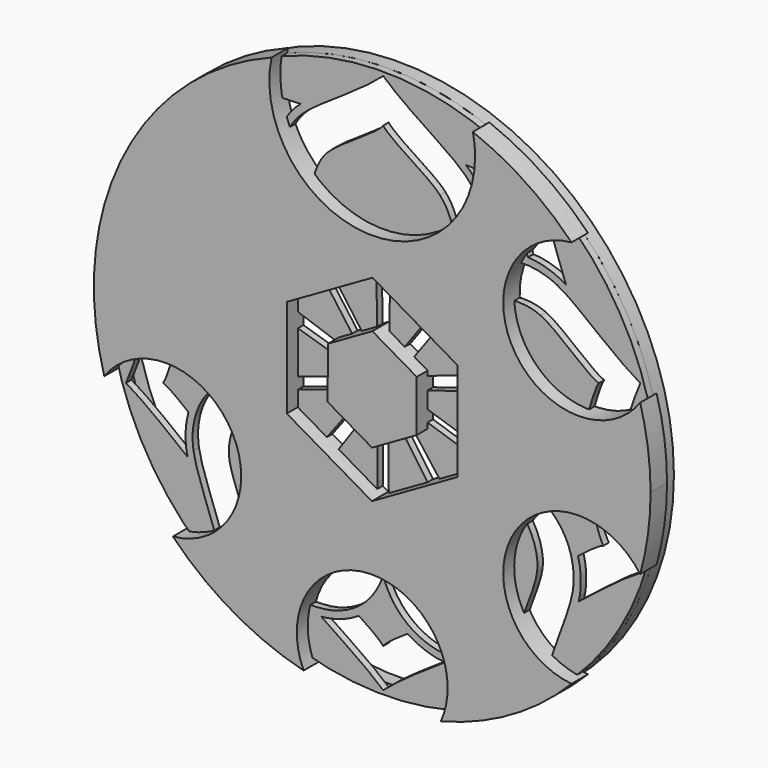
from build123d import *

# Parameters (mm, degrees)
F0_R     = 40
F1_DEPTH = 1
F2_R     = 40
F3_DEPTH = 2
F4_T     = -1
F6_DEPTH = 3


with BuildPart() as f1:
    # F0 (on Front) → F1 (new body)
    with BuildSketch(Plane.XZ):
        Circle(F0_R)
        with BuildLine():
            add(Edge.make_bspline(
                [(3.5534648058, -31.0212486438), (5.4467639917, -32.2635820829), (7.3085112664, -32.6879645142), (8.144360142, -32.8156482718)],
                knots=[0, 0, 0, 0, 1, 1, 1, 1], degree=3))
            add(Edge.make_bspline(
                [(8.144360142, -32.8156482718), (8.4174410108, -32.8579020009), (8.7100803743, -32.889269398), (9.012129957, -32.9147323438)],
                knots=[0, 0, 0, 0, 1, 1, 1, 1], degree=3))
            add(Edge.make_bspline(
                [(9.012129957, -32.9147323438), (6.2822438391, -34.821316545), (2.7349602557, -36.9727509576), (-0.0059967083, -39.430109749)],
                knots=[0, 0, 0, 0, 1, 1, 1, 1], degree=3))
            add(Edge.make_bspline(
                [(-0.0059967083, -39.430109749), (-2.7493523555, -36.969798732), (-6.3001417068, -34.8165191784), (-9.0315039375, -32.9086433785)],
                knots=[0, 0, 0, 0, 1, 1, 1, 1], degree=3))
            add(Edge.make_bspline(
                [(-9.0315039375, -32.9086433785), (-8.7255795588, -32.8831804326), (-8.4292499133, -32.8518130356), (-8.153585847, -32.8099283347)],
                knots=[0, 0, 0, 0, 1, 1, 1, 1], degree=3))
            Line((-8.153585847, -32.8099283347), (-8.1548774457, -32.8093747924))
            add(Edge.make_bspline(
                [(-8.1548774457, -32.8093747924), (-7.3169989151, -32.6818755489), (-5.4502697596, -32.2654272239), (-3.5521732071, -31.0286292078)],
                knots=[0, 0, 0, 0, 1, 1, 1, 1], degree=3))
            add(Edge.make_bspline(
                [(-3.5521732071, -31.0286292078), (-2.0007786495, -32.048992184), (-0.5704253419, -33.0138164159), (-0.0059967083, -33.7646042911)],
                knots=[0, 0, 0, 0, 1, 1, 1, 1], degree=3))
            add(Edge.make_bspline(
                [(-0.0059967083, -33.7646042911), (0.5611996369, -33.0114177325), (1.996165797, -32.0441948174), (3.5534648058, -31.0212486438)],
                knots=[0, 0, 0, 0, 1, 1, 1, 1], degree=3))
        make_face(mode=Mode.SUBTRACT)
        with BuildLine():
            add(Edge.make_bspline(
                [(-28.4049309548, -12.9656213328), (-29.0009114997, -15.1502682835), (-28.8293133861, -17.0520551181), (-28.6925884376, -17.8864278808)],
                knots=[0, 0, 0, 0, 1, 1, 1, 1], degree=3))
            add(Edge.make_bspline(
                [(-28.6925884376, -17.8864278808), (-28.649227624, -18.1589552074), (-28.5875999144, -18.4467972042), (-28.5185916408, -18.7416507369)],
                knots=[0, 0, 0, 0, 1, 1, 1, 1], degree=3))
            add(Edge.make_bspline(
                [(-28.5185916408, -18.7416507369), (-31.1759637171, -16.7352444074), (-34.3184233639, -14.026577411), (-37.501845141, -12.1792222362)],
                knots=[0, 0, 0, 0, 1, 1, 1, 1], degree=3))
            add(Edge.make_bspline(
                [(-37.501845141, -12.1792222362), (-36.0098641238, -8.8094412175), (-35.0594319918, -4.76655276), (-34.0887033087, -1.5801787573)],
                knots=[0, 0, 0, 0, 1, 1, 1, 1], degree=3))
            add(Edge.make_bspline(
                [(-34.0887033087, -1.5801787573), (-33.970060742, -1.8630388734), (-33.8492040062, -2.1350126577), (-33.7235499037, -2.3841066934)],
                knots=[0, 0, 0, 0, 1, 1, 1, 1], degree=3))
            Line((-33.7235499037, -2.3841066934), (-33.7235499037, -2.3835531511))
            add(Edge.make_bspline(
                [(-33.7235499037, -2.3835531511), (-33.3438198847, -3.1398764494), (-32.3706925183, -4.7870338251), (-30.6078448015, -6.2094530264)],
                knots=[0, 0, 0, 0, 1, 1, 1, 1], degree=3))
            add(Edge.make_bspline(
                [(-30.6078448015, -6.2094530264), (-31.098652309, -8.001269457), (-31.5739606321, -9.6589441365), (-32.1142179185, -10.42855245)],
                knots=[0, 0, 0, 0, 1, 1, 1, 1], degree=3))
            add(Edge.make_bspline(
                [(-32.1142179185, -10.42855245), (-31.2219077282, -10.735030371), (-29.8594556096, -11.8005993018), (-28.4049309548, -12.9656213328)],
                knots=[0, 0, 0, 0, 1, 1, 1, 1], degree=3))
        make_face(mode=Mode.SUBTRACT)
        with BuildLine():
            add(Edge.make_bspline(
                [(30.6010177798, -6.2065008008), (32.368293835, -4.7901705648), (33.3465875962, -3.1500247249), (33.7261331011, -2.3951775395)],
                knots=[0, 0, 0, 0, 1, 1, 1, 1], degree=3))
            add(Edge.make_bspline(
                [(33.7261331011, -2.3951775395), (33.8508646331, -2.148482187), (33.9715368548, -1.8800141707), (34.0887033087, -1.6001062801)],
                knots=[0, 0, 0, 0, 1, 1, 1, 1], degree=3))
            add(Edge.make_bspline(
                [(34.0887033087, -1.6001062801), (35.0585094213, -4.7853731982), (36.0087570392, -8.8240178314), (37.498154859, -12.189924054)],
                knots=[0, 0, 0, 0, 1, 1, 1, 1], degree=3))
            add(Edge.make_bspline(
                [(37.498154859, -12.189924054), (34.3114118281, -14.0385708276), (31.1652618993, -16.75111262), (28.5067827383, -18.7580724919)],
                knots=[0, 0, 0, 0, 1, 1, 1, 1], degree=3))
            add(Edge.make_bspline(
                [(28.5067827383, -18.7580724919), (28.5767135825, -18.4600822195), (28.6387103202, -18.1687344547), (28.6844698172, -17.8936239307)],
                knots=[0, 0, 0, 0, 1, 1, 1, 1], degree=3))
            Line((28.6844698172, -17.8936239307), (28.6833627326, -17.8936239307))
            add(Edge.make_bspline(
                [(28.6833627326, -17.8936239307), (28.8210102516, -17.0581440834), (29.0022030984, -15.1539585655), (28.4123115188, -12.9669129315)],
                knots=[0, 0, 0, 0, 1, 1, 1, 1], degree=3))
            add(Edge.make_bspline(
                [(28.4123115188, -12.9669129315), (29.8622233211, -11.8061347248), (31.2222767564, -10.7444405901), (32.1108966647, -10.4387007255)],
                knots=[0, 0, 0, 0, 1, 1, 1, 1], degree=3))
            add(Edge.make_bspline(
                [(32.1108966647, -10.4387007255), (31.5693477796, -9.6674317851), (31.0929323719, -8.0036681403), (30.6010177798, -6.2065008008)],
                knots=[0, 0, 0, 0, 1, 1, 1, 1], degree=3))
        make_face(mode=Mode.SUBTRACT)
        with BuildLine():
            add(Edge.make_bspline(
                [(-21.108505362, 23.0079857703), (-23.3706482349, 22.9004140496), (-25.12666893, 22.1494416603), (-25.8781948617, 21.761777535)],
                knots=[0, 0, 0, 0, 1, 1, 1, 1], degree=3))
            add(Edge.make_bspline(
                [(-25.8781948617, 21.761777535), (-26.1235986154, 21.6355698903), (-26.3780435601, 21.488327638), (-26.6374703855, 21.3316751666)],
                knots=[0, 0, 0, 0, 1, 1, 1, 1], degree=3))
            add(Edge.make_bspline(
                [(-26.6374703855, 21.3316751666), (-25.5497597626, 24.4785631518), (-23.9448561159, 28.3039094848), (-23.1717420345, 31.9028570163)],
                knots=[0, 0, 0, 0, 1, 1, 1, 1], degree=3))
            add(Edge.make_bspline(
                [(-23.1717420345, 31.9028570163), (-19.5063694268, 31.5257101948), (-15.3680871792, 31.871120591), (-12.0370541217, 31.9325637865)],
                knots=[0, 0, 0, 0, 1, 1, 1, 1], degree=3))
            add(Edge.make_bspline(
                [(-12.0370541217, 31.9325637865), (-12.2691728602, 31.7319969592), (-12.4904052668, 31.5329062447), (-12.6887579249, 31.3367677558)],
                knots=[0, 0, 0, 0, 1, 1, 1, 1], degree=3))
            Line((-12.6887579249, 31.3367677558), (-12.6880198685, 31.3367677558))
            add(Edge.make_bspline(
                [(-12.6880198685, 31.3367677558), (-13.2897203504, 30.7415252674), (-14.5560406226, 29.307850706), (-15.3643968972, 27.1912894583)],
                knots=[0, 0, 0, 0, 1, 1, 1, 1], degree=3))
            add(Edge.make_bspline(
                [(-15.3643968972, 27.1912894583), (-17.2202397207, 27.1041988029), (-18.9430478777, 27.0440472061), (-19.8420005757, 27.3197112723)],
                knots=[0, 0, 0, 0, 1, 1, 1, 1], degree=3))
            add(Edge.make_bspline(
                [(-19.8420005757, 27.3197112723), (-19.8576842742, 26.3773977607), (-20.4501590512, 24.7510904783), (-21.108505362, 23.0079857703)],
                knots=[0, 0, 0, 0, 1, 1, 1, 1], degree=3))
        make_face(mode=Mode.SUBTRACT)
        with BuildLine():
            add(Edge.make_bspline(
                [(25.3995652848, 20.8154047132), (23.1233993402, 21.989283421), (18.8856639924, 23.0513465839), (14.5558561085, 20.0171967142)],
                knots=[0, 0, 0, 0, 1, 1, 1, 1], degree=3))
            add(Edge.make_bspline(
                [(37.501845141, 12.1797757785), (32.94988228, 14.8203570717), (28.4811352784, 19.2258157368), (25.3995652848, 20.8154047132)],
                knots=[0, 0, 0, 0, 1, 1, 1, 1], degree=3))
            add(Edge.make_bspline(
                [(32.786587301, -1.920976301), (34.3457314508, 1.1764619052), (35.3723679064, 7.368201578), (37.501845141, 12.1797757785)],
                knots=[0, 0, 0, 0, 1, 1, 1, 1], degree=3))
            add(Edge.make_bspline(
                [(23.5446450318, -7.6482939826), (28.8315275553, -7.5575130451), (31.6352193135, -4.2074750352), (32.786587301, -1.920976301)],
                knots=[0, 0, 0, 0, 1, 1, 1, 1], degree=3))
            add(Edge.make_bspline(
                [(23.5151227757, -7.6458952993), (23.523056882, -7.6458952993), (23.5374489819, -7.6482939826), (23.5446450318, -7.6482939826)],
                knots=[0, 0, 0, 0, 1, 1, 1, 1], degree=3))
            add(Edge.make_bspline(
                [(23.5354193267, -7.6578887159), (23.5309909883, -7.6541984338), (23.5202891705, -7.6494010672), (23.5151227757, -7.6458952993)],
                knots=[0, 0, 0, 0, 1, 1, 1, 1], degree=3))
            add(Edge.make_bspline(
                [(27.6451018887, -17.7244245005), (28.0580444458, -15.1962122945), (27.7589470887, -10.8381737532), (23.5354193267, -7.6578887159)],
                knots=[0, 0, 0, 0, 1, 1, 1, 1], degree=3))
            add(Edge.make_bspline(
                [(23.1717420345, -31.9026725022), (24.2769814969, -26.757681322), (27.0862086781, -21.1460539814), (27.6451018887, -17.7244245005)],
                knots=[0, 0, 0, 0, 1, 1, 1, 1], degree=3))
            add(Edge.make_bspline(
                [(8.3043338672, -31.775726801), (11.7326058557, -32.3012229595), (17.9379995719, -31.3635223004), (23.1717420345, -31.9026725022)],
                knots=[0, 0, 0, 0, 1, 1, 1, 1], degree=3))
            add(Edge.make_bspline(
                [(0.0011993417, -24.756072359), (1.7212397871, -29.7554819139), (5.7737229779, -31.3871401052), (8.3043338672, -31.775726801)],
                knots=[0, 0, 0, 0, 1, 1, 1, 1], degree=3))
            add(Edge.make_bspline(
                [(-0.005443166, -24.7271036453), (-0.0028599686, -24.7342996952), (-0.0010148276, -24.7488763091), (0.0011993417, -24.756072359)],
                knots=[0, 0, 0, 0, 1, 1, 1, 1], degree=3))
            add(Edge.make_bspline(
                [(-0.0100560185, -24.7494298514), (-0.0083953916, -24.7440789425), (-0.007288307, -24.7331926106), (-0.005443166, -24.7271036453)],
                knots=[0, 0, 0, 0, 1, 1, 1, 1], degree=3))
            add(Edge.make_bspline(
                [(-8.3137440863, -31.7690842934), (-5.7825796547, -31.3803130835), (-1.730096464, -29.7495774627), (-0.0100560185, -24.7494298514)],
                knots=[0, 0, 0, 0, 1, 1, 1, 1], degree=3))
            add(Edge.make_bspline(
                [(-23.1805987114, -31.8954764523), (-17.9461181924, -31.3574333351), (-11.7414625326, -32.2943959377), (-8.3137440863, -31.7690842934)],
                knots=[0, 0, 0, 0, 1, 1, 1, 1], degree=3))
            add(Edge.make_bspline(
                [(-27.6543275937, -17.7172284506), (-27.0948808408, -21.139780502), (-24.2858381738, -26.7515923567), (-23.1805987114, -31.8954764523)],
                knots=[0, 0, 0, 0, 1, 1, 1, 1], degree=3))
            add(Edge.make_bspline(
                [(-23.5440914895, -7.6506926659), (-27.7678037656, -10.8315312456), (-28.0670856367, -15.1901233292), (-27.6543275937, -17.7172284506)],
                knots=[0, 0, 0, 0, 1, 1, 1, 1], degree=3))
            add(Edge.make_bspline(
                [(-23.5186285436, -7.636116052), (-23.5247175089, -7.6403598763), (-23.5385560665, -7.6470023839), (-23.5440914895, -7.6506926659)],
                knots=[0, 0, 0, 0, 1, 1, 1, 1], degree=3))
            add(Edge.make_bspline(
                [(-23.5415082921, -7.6381457071), (-23.5361573831, -7.6381457071), (-23.5247175089, -7.636116052), (-23.5186285436, -7.636116052)],
                knots=[0, 0, 0, 0, 1, 1, 1, 1], degree=3))
            add(Edge.make_bspline(
                [(-32.7834505613, -1.9102744832), (-31.6318980596, -4.1976957879), (-28.8282063015, -7.5479183119), (-23.5415082921, -7.6381457071)],
                knots=[0, 0, 0, 0, 1, 1, 1, 1], degree=3))
            add(Edge.make_bspline(
                [(-37.498154859, 12.189924054), (-35.3684931102, 7.3785343676), (-34.3425947111, 1.1873482372), (-32.7834505613, -1.9102744832)],
                knots=[0, 0, 0, 0, 1, 1, 1, 1], degree=3))
            add(Edge.make_bspline(
                [(-25.3956904887, 20.8261065311), (-28.4779985386, 19.2365175547), (-32.9472990826, 14.8308743754), (-37.498154859, 12.189924054)],
                knots=[0, 0, 0, 0, 1, 1, 1, 1], degree=3))
            add(Edge.make_bspline(
                [(-14.5525348547, 20.027898532), (-18.8825272527, 23.0618638876), (-23.1202626005, 21.9996162107), (-25.3956904887, 20.8261065311)],
                knots=[0, 0, 0, 0, 1, 1, 1, 1], degree=3))
            add(Edge.make_bspline(
                [(-14.5302086485, 20.007786495), (-14.5361130998, 20.0127683758), (-14.5464458894, 20.0234701936), (-14.5525348547, 20.027898532)],
                knots=[0, 0, 0, 0, 1, 1, 1, 1], degree=3))
            add(Edge.make_bspline(
                [(-14.5392498395, 20.0293746448), (-14.5374046985, 20.0238392218), (-14.5318692754, 20.0136909463), (-14.5302086485, 20.007786495)],
                knots=[0, 0, 0, 0, 1, 1, 1, 1], degree=3))
            add(Edge.make_bspline(
                [(-11.947749297, 30.5887475921), (-13.7672428427, 28.7867828859), (-16.0867696009, 25.0848764863), (-14.5392498395, 20.0293746448)],
                knots=[0, 0, 0, 0, 1, 1, 1, 1], degree=3))
            add(Edge.make_bspline(
                [(0.0056276801, 39.430109749), (-3.9123447314, 35.9178838447), (-9.4835634839, 33.0289465721), (-11.947749297, 30.5887475921)],
                knots=[0, 0, 0, 0, 1, 1, 1, 1], degree=3))
            add(Edge.make_bspline(
                [(11.9584511148, 30.5887475921), (9.49463433, 33.0289465721), (3.9236000915, 35.9178838447), (0.0056276801, 39.430109749)],
                knots=[0, 0, 0, 0, 1, 1, 1, 1], degree=3))
            add(Edge.make_bspline(
                [(14.5503206855, 20.0293746448), (16.097840447, 25.0848764863), (13.7781291746, 28.7867828859), (11.9584511148, 30.5887475921)],
                knots=[0, 0, 0, 0, 1, 1, 1, 1], degree=3))
            add(Edge.make_bspline(
                [(14.5388808113, 20.0020665579), (14.5409104664, 20.009631636), (14.5486600586, 20.022363109), (14.5503206855, 20.0293746448)],
                knots=[0, 0, 0, 0, 1, 1, 1, 1], degree=3))
            add(Edge.make_bspline(
                [(14.5558561085, 20.0171967142), (14.5506897137, 20.0138754604), (14.5434936638, 20.0057568399), (14.5388808113, 20.0020665579)],
                knots=[0, 0, 0, 0, 1, 1, 1, 1], degree=3))
        make_face(mode=Mode.SUBTRACT)
        with BuildLine():
            add(Edge.make_bspline(
                [(15.3583079319, 27.1853850071), (14.5578857636, 29.3041604239), (13.3006066824, 30.7409717251), (12.6998287709, 31.3356606712)],
                knots=[0, 0, 0, 0, 1, 1, 1, 1], degree=3))
            add(Edge.make_bspline(
                [(12.6998287709, 31.3356606712), (12.5038747961, 31.5299540191), (12.2865171856, 31.727937649), (12.0555055317, 31.9259212789)],
                knots=[0, 0, 0, 0, 1, 1, 1, 1], degree=3))
            add(Edge.make_bspline(
                [(12.0555055317, 31.9259212789), (15.3850624765, 31.8639245411), (19.5200234702, 31.5196212295), (23.1811522537, 31.8962145087)],
                knots=[0, 0, 0, 0, 1, 1, 1, 1], degree=3))
            add(Edge.make_bspline(
                [(23.1811522537, 31.8962145087), (23.9548198773, 28.2939457233), (25.561384151, 24.4638020238), (26.6496483161, 21.3150688976)],
                knots=[0, 0, 0, 0, 1, 1, 1, 1], degree=3))
            add(Edge.make_bspline(
                [(26.6496483161, 21.3150688976), (26.3874537792, 21.4739355382), (26.1296875807, 21.6224693891), (25.8817006296, 21.7512602313)],
                knots=[0, 0, 0, 0, 1, 1, 1, 1], degree=3))
            Line((25.8817006296, 21.7512602313), (25.8817006296, 21.7501531467))
            add(Edge.make_bspline(
                [(25.8817006296, 21.7501531467), (25.1299901839, 22.1392933848), (23.374338517, 22.9000450214), (21.112195644, 23.0149973061)],
                knots=[0, 0, 0, 0, 1, 1, 1, 1], degree=3))
            add(Edge.make_bspline(
                [(21.112195644, 23.0149973061), (20.4558789883, 24.752382077), (19.8670944934, 26.3737074787), (19.8512262807, 27.3138068211)],
                knots=[0, 0, 0, 0, 1, 1, 1, 1], degree=3))
            add(Edge.make_bspline(
                [(19.8512262807, 27.3138068211), (18.949136843, 27.0368511562), (17.2204242348, 27.0979253235), (15.3583079319, 27.1853850071)],
                knots=[0, 0, 0, 0, 1, 1, 1, 1], degree=3))
        make_face(mode=Mode.SUBTRACT)
    extrude(amount=F1_DEPTH)


with BuildPart() as f1b:
    # F0 (on Front) → F1, piece 2 (new body)
    with BuildSketch(Plane.XZ):
        with BuildLine():
            add(Edge.make_bspline(
                [(31.4464613886, 10.2117483818), (30.291403119, 8.564591006), (29.4315674104, 2.8594150165), (28.0847989903, 0.4461550952)],
                knots=[0, 0, 0, 0, 1, 1, 1, 1], degree=3))
            add(Edge.make_bspline(
                [(22.9857518212, 16.1370496933), (25.4955126171, 14.9759024585), (29.5439364976, 10.8654818401), (31.4464613886, 10.2117483818)],
                knots=[0, 0, 0, 0, 1, 1, 1, 1], degree=3))
            add(Edge.make_bspline(
                [(8.3218627067, 10.07262475), (13.5153810954, 17.1295510403), (19.7831405776, 17.6203585478), (22.9857518212, 16.1370496933)],
                knots=[0, 0, 0, 0, 1, 1, 1, 1], degree=3))
            Line((8.3218627067, 10.07262475), (3.9130827878, 4.0224073924))
            add(Edge.make_bspline(
                [(2.6249898517, 4.9621377066), (3.0990065761, 4.7108295016), (3.5316921419, 4.3934652486), (3.9130827878, 4.0224073924)],
                knots=[0, 0, 0, 0, 1, 1, 1, 1], degree=3))
            Line((2.6249898517, 4.9621377066), (7.0184551003, 11.0278542486))
            add(Edge.make_bspline(
                [(8.2548840882, 26.8480932313), (10.6554125366, 24.2593604003), (12.1254363758, 18.1465927626), (7.0184551003, 11.0278542486)],
                knots=[0, 0, 0, 0, 1, 1, 1, 1], degree=3))
            add(Edge.make_bspline(
                [(0.0056276801, 33.0632661948), (1.2153021234, 31.4555948366), (6.3752389458, 28.874980626), (8.2548840882, 26.8480932313)],
                knots=[0, 0, 0, 0, 1, 1, 1, 1], degree=3))
            add(Edge.make_bspline(
                [(-8.2436287281, 26.8480932313), (-6.3643526138, 28.874980626), (-1.2040467633, 31.4555948366), (0.0056276801, 33.0632661948)],
                knots=[0, 0, 0, 0, 1, 1, 1, 1], degree=3))
            add(Edge.make_bspline(
                [(-7.0073842543, 11.0278542486), (-12.1145500439, 18.1465927626), (-10.6441571765, 24.2593604003), (-8.2436287281, 26.8480932313)],
                knots=[0, 0, 0, 0, 1, 1, 1, 1], degree=3))
            Line((-7.0073842543, 11.0278542486), (-2.6155796326, 4.9643518758))
            add(Edge.make_bspline(
                [(-3.9051486815, 4.0264667026), (-3.5230199792, 4.3967865024), (-3.0903344134, 4.7135972131), (-2.6155796326, 4.9643518758)],
                knots=[0, 0, 0, 0, 1, 1, 1, 1], degree=3))
            Line((-3.9051486815, 4.0264667026), (-8.3194640234, 10.0827730255))
            add(Edge.make_bspline(
                [(-22.9829841096, 16.1475669971), (-19.7790812674, 17.6306913374), (-13.5115062993, 17.1398838299), (-8.3194640234, 10.0827730255)],
                knots=[0, 0, 0, 0, 1, 1, 1, 1], degree=3))
            add(Edge.make_bspline(
                [(-31.4433246489, 10.2224501996), (-29.5402462156, 10.876183658), (-25.4912687928, 14.9864197622), (-22.9829841096, 16.1475669971)],
                knots=[0, 0, 0, 0, 1, 1, 1, 1], degree=3))
            add(Edge.make_bspline(
                [(-28.0809241942, 0.4564878848), (-29.4284306707, 2.8703013484), (-30.2880818652, 8.5751083098), (-31.4433246489, 10.2224501996)],
                knots=[0, 0, 0, 0, 1, 1, 1, 1], degree=3))
            add(Edge.make_bspline(
                [(-12.6531467035, -3.2570429032), (-21.002040726, -5.9138614373), (-26.3610682628, -2.6263737075), (-28.0809241942, 0.4564878848)],
                knots=[0, 0, 0, 0, 1, 1, 1, 1], degree=3))
            Line((-12.6531467035, -3.2570429032), (-5.5283192242, -0.9531998435))
            add(Edge.make_bspline(
                [(-5.0343749769, -2.4693522079), (-5.2676008001, -1.9966270822), (-5.4356931457, -1.4881062211), (-5.5283192242, -0.9531998435)],
                knots=[0, 0, 0, 0, 1, 1, 1, 1], degree=3))
            Line((-5.0343749769, -2.4693522079), (-12.160494055, -4.7960750161))
            add(Edge.make_bspline(
                [(-22.458964064, -16.8682790739), (-22.8798407274, -13.3626956772), (-20.4759910252, -7.5540072772), (-12.160494055, -4.7960750161)],
                knots=[0, 0, 0, 0, 1, 1, 1, 1], degree=3))
            add(Edge.make_bspline(
                [(-19.4388372659, -26.7449498491), (-19.472049804, -24.7331926106), (-22.1301599368, -19.6121882634), (-22.458964064, -16.8682790739)],
                knots=[0, 0, 0, 0, 1, 1, 1, 1], degree=3))
            add(Edge.make_bspline(
                [(-9.111214029, -26.5654176292), (-11.8237558214, -27.1010620632), (-17.5150932534, -26.1556118119), (-19.4388372659, -26.7449498491)],
                knots=[0, 0, 0, 0, 1, 1, 1, 1], degree=3))
            add(Edge.make_bspline(
                [(-0.8123233277, -13.0399805153), (-0.8656479028, -21.8010790385), (-5.6478843613, -25.8823464289), (-9.111214029, -26.5654176292)],
                knots=[0, 0, 0, 0, 1, 1, 1, 1], degree=3))
            Line((-0.8123233277, -13.0399805153), (-0.8014369958, -5.549999631))
            add(Edge.make_bspline(
                [(0.0048896237, -5.6147640803), (-0.269667358, -5.6147640803), (-0.5379508602, -5.5880095357), (-0.8014369958, -5.549999631)],
                knots=[0, 0, 0, 0, 1, 1, 1, 1], degree=3))
            add(Edge.make_bspline(
                [(0.792580319, -5.5523983143), (0.5344450923, -5.5893011344), (0.2731731259, -5.6147640803), (0.0048896237, -5.6147640803)],
                knots=[0, 0, 0, 0, 1, 1, 1, 1], degree=3))
            Line((0.792580319, -5.5523983143), (0.8032821368, -13.0471765652))
            add(Edge.make_bspline(
                [(9.1029108945, -26.5720601368), (5.6384741422, -25.8889889365), (0.856791226, -21.8084596025), (0.8032821368, -13.0471765652)],
                knots=[0, 0, 0, 0, 1, 1, 1, 1], degree=3))
            add(Edge.make_bspline(
                [(19.4292425327, -26.752145899), (17.5058675484, -26.1622543195), (11.8139765741, -27.1077045708), (9.1029108945, -26.5720601368)],
                knots=[0, 0, 0, 0, 1, 1, 1, 1], degree=3))
            add(Edge.make_bspline(
                [(22.4499228731, -16.8743680392), (22.12130326, -19.6195688274), (19.4630086131, -24.7403886605), (19.4292425327, -26.752145899)],
                knots=[0, 0, 0, 0, 1, 1, 1, 1], degree=3))
            add(Edge.make_bspline(
                [(12.1508993217, -4.8023484955), (20.4671343484, -7.5600962426), (22.8707995365, -13.3693381848), (22.4499228731, -16.8743680392)],
                knots=[0, 0, 0, 0, 1, 1, 1, 1], degree=3))
            Line((12.1508993217, -4.8023484955), (5.0312382372, -2.4778398565))
            add(Edge.make_bspline(
                [(5.5272121396, -0.9616874922), (5.4342170329, -1.4973319261), (5.2648330885, -2.0056682732), (5.0312382372, -2.4778398565)],
                knots=[0, 0, 0, 0, 1, 1, 1, 1], degree=3))
            Line((5.5272121396, -0.9616874922), (12.6570214996, -3.2673756929))
            add(Edge.make_bspline(
                [(28.0847989903, 0.4461550952), (26.3643895166, -2.6374445535), (21.0059155221, -5.9240097128), (12.6570214996, -3.2673756929)],
                knots=[0, 0, 0, 0, 1, 1, 1, 1], degree=3))
        make_face()
        with BuildLine():
            add(Edge.make_bspline(
                [(-3.9533068617, -3.9783085223), (-3.7527400344, -4.1783218074), (-3.5399952764, -4.3694784155), (-3.3041862559, -4.5399694445)],
                knots=[0, 0, 0, 0, 1, 1, 1, 1], degree=3))
            add(Edge.make_bspline(
                [(-3.3041862559, -4.5399694445), (-3.0696688341, -4.7102759593), (-2.8242650803, -4.8536434154), (-2.5727723613, -4.9822497435)],
                knots=[0, 0, 0, 0, 1, 1, 1, 1], degree=3))
            Line((-2.5727723613, -4.9822497435), (-7.2359972249, -11.6563092752))
            add(Edge.make_bspline(
                [(-7.2359972249, -11.6563092752), (-7.5624026688, -12.1059701382), (-8.1923338081, -12.2068993512), (-8.6432862699, -11.8786487663)],
                knots=[0, 0, 0, 0, 1, 1, 1, 1], degree=3))
            add(Edge.make_bspline(
                [(-8.6432862699, -11.8786487663), (-9.0942387317, -11.5516897801), (-9.1935073178, -10.9223121831), (-8.8656257611, -10.4719132636)],
                knots=[0, 0, 0, 0, 1, 1, 1, 1], degree=3))
            Line((-8.8656257611, -10.4719132636), (-3.9533068617, -3.9783085223))
        make_face(mode=Mode.SUBTRACT)
        with BuildLine():
            add(Edge.make_bspline(
                [(2.5620705434, -4.9896303075), (2.8135632625, -4.8602859231), (3.0615502137, -4.7174720092), (3.2971747201, -4.5458738957)],
                knots=[0, 0, 0, 0, 1, 1, 1, 1], degree=3))
            add(Edge.make_bspline(
                [(3.2971747201, -4.5458738957), (3.5316921419, -4.3740912681), (3.7433298153, -4.1857023714), (3.9440811567, -3.9866116569)],
                knots=[0, 0, 0, 0, 1, 1, 1, 1], degree=3))
            Line((3.9440811567, -3.9866116569), (8.8503110908, -10.4835376519))
            add(Edge.make_bspline(
                [(8.8503110908, -10.4835376519), (9.1767165347, -10.933198515), (9.0776324627, -11.5636831967), (8.6264954868, -11.8913802393)],
                knots=[0, 0, 0, 0, 1, 1, 1, 1], degree=3))
            add(Edge.make_bspline(
                [(8.6264954868, -11.8913802393), (8.175543025, -12.2185237396), (7.5467189703, -12.1181480689), (7.2192064418, -11.6683026917)],
                knots=[0, 0, 0, 0, 1, 1, 1, 1], degree=3))
            Line((7.2192064418, -11.6683026917), (2.5620705434, -4.9896303075))
        make_face(mode=Mode.SUBTRACT)
        with BuildLine():
            add(Edge.make_bspline(
                [(-5.0054062631, 2.5313489457), (-5.1334590489, 2.2783801138), (-5.2495184182, 2.0169236333), (-5.339007757, 1.7399679684)],
                knots=[0, 0, 0, 0, 1, 1, 1, 1], degree=3))
            add(Edge.make_bspline(
                [(-5.339007757, 1.7399679684), (-5.4284970957, 1.4635658457), (-5.4890177207, 1.1862411525), (-5.5336701331, 0.9076248607)],
                knots=[0, 0, 0, 0, 1, 1, 1, 1], degree=3))
            Line((-5.5336701331, 0.9076248607), (-13.3210877475, 3.2799226517))
            add(Edge.make_bspline(
                [(-13.3210877475, 3.2799226517), (-13.8506432162, 3.4518897934), (-14.1406993822, 4.0196396809), (-13.9691012687, 4.5497486918)],
                knots=[0, 0, 0, 0, 1, 1, 1, 1], degree=3))
            add(Edge.make_bspline(
                [(-13.9691012687, 4.5497486918), (-13.7962115565, 5.0793041604), (-13.2291997254, 5.3682532419), (-12.6996442568, 5.1962861002)],
                knots=[0, 0, 0, 0, 1, 1, 1, 1], degree=3))
            Line((-12.6996442568, 5.1962861002), (-5.0054062631, 2.5313489457))
        make_face(mode=Mode.SUBTRACT)
        with BuildLine():
            add(Edge.make_bspline(
                [(0.0048896237, 5.0888988937), (2.8124561779, 5.0888988937), (5.0897292071, 2.8105187798), (5.0897292071, 0.003690282)],
                knots=[0, 0, 0, 0, 1, 1, 1, 1], degree=3))
            add(Edge.make_bspline(
                [(5.0897292071, 0.003690282), (5.0897292071, -2.810887808), (2.8124561779, -5.0881608373), (0.0048896237, -5.0881608373)],
                knots=[0, 0, 0, 0, 1, 1, 1, 1], degree=3))
            add(Edge.make_bspline(
                [(0.0048896237, -5.0881608373), (-2.8109800651, -5.0881608373), (-5.0893601789, -2.810887808), (-5.0893601789, 0.003690282)],
                knots=[0, 0, 0, 0, 1, 1, 1, 1], degree=3))
            add(Edge.make_bspline(
                [(-5.0893601789, 0.003690282), (-5.0893601789, 2.8105187798), (-2.8109800651, 5.0888988937), (0.0048896237, 5.0888988937)],
                knots=[0, 0, 0, 0, 1, 1, 1, 1], degree=3))
        make_face(mode=Mode.SUBTRACT)
        with BuildLine():
            add(Edge.make_bspline(
                [(5.5373604151, 0.8947088737), (5.4916009181, 1.1740632219), (5.4323718919, 1.4534175702), (5.342698039, 1.7314803197)],
                knots=[0, 0, 0, 0, 1, 1, 1, 1], degree=3))
            add(Edge.make_bspline(
                [(5.342698039, 1.7314803197), (5.2522861297, 2.007144386), (5.1373338451, 2.2667557255), (5.0103881439, 2.519171015)],
                knots=[0, 0, 0, 0, 1, 1, 1, 1], degree=3))
            Line((5.0103881439, 2.519171015), (12.7044416234, 5.1774656619))
            add(Edge.make_bspline(
                [(12.7044416234, 5.1774656619), (13.2341816062, 5.3492482896), (13.8035921205, 5.0599301799), (13.975190234, 4.5298211689)],
                knots=[0, 0, 0, 0, 1, 1, 1, 1], degree=3))
            add(Edge.make_bspline(
                [(13.975190234, 4.5298211689), (14.1471573758, 3.9998966721), (13.8569166956, 3.4328848411), (13.3282837974, 3.260364157)],
                knots=[0, 0, 0, 0, 1, 1, 1, 1], degree=3))
            Line((13.3282837974, 3.260364157), (5.5373604151, 0.8947088737))
        make_face(mode=Mode.SUBTRACT)
        with BuildLine():
            add(Edge.make_bspline(
                [(0.8602969939, 5.5433571234), (0.5802045892, 5.5861643947), (0.2962373885, 5.6153176226), (0.0048896237, 5.6153176226)],
                knots=[0, 0, 0, 0, 1, 1, 1, 1], degree=3))
            add(Edge.make_bspline(
                [(0.0048896237, 5.6153176226), (-0.2851665424, 5.6153176226), (-0.5682111727, 5.5863489088), (-0.8473810069, 5.5439106657)],
                knots=[0, 0, 0, 0, 1, 1, 1, 1], degree=3))
            Line((-0.8473810069, 5.5439106657), (-0.9973909706, 13.683381184))
            add(Edge.make_bspline(
                [(-0.9973909706, 13.683381184), (-0.9973909706, 14.2402447395), (-0.5469920511, 14.6911972013), (0.0104250467, 14.6911972013)],
                knots=[0, 0, 0, 0, 1, 1, 1, 1], degree=3))
            add(Edge.make_bspline(
                [(0.0104250467, 14.6911972013), (0.5672886022, 14.6911972013), (1.0175030076, 14.2402447395), (1.0175030076, 13.683381184)],
                knots=[0, 0, 0, 0, 1, 1, 1, 1], degree=3))
            Line((1.0175030076, 13.683381184), (0.8602969939, 5.5433571234))
        make_face(mode=Mode.SUBTRACT)
    extrude(amount=F1_DEPTH)


with BuildPart() as f3:
    # F2 (on Front) → F3 (new body)
    with BuildSketch(Plane.XZ):
        Circle(F2_R)
    extrude(amount=-F3_DEPTH)

    # F4
    f4_openings = [f3.faces().sort_by_distance(p)[0] for p in [
        (0, 2, 0),
        (0, 0, 0),
    ]]
    offset(amount=F4_T, openings=f4_openings)

    # F5 (on Front) → F6 (join)
    with BuildSketch(Plane.XZ):
        with BuildLine():
            ThreePointArc((29.0693669356, 28.3318343404), (22.3856605229, 33.8615288208), (14.6796276557, 37.8448076097))
            ThreePointArc((14.6796276557, 37.8448076097), (14.9196916834, 36.3113120447), (14.9999996647, 34.7612184947))
            ThreePointArc((14.9999996647, 34.7612184947), (-1.55009355, 19.8415268113), (-14.6796276557, 37.8448076097))
            ThreePointArc((-14.6796276557, 37.8448076097), (-22.3856605228, 33.8615288209), (-29.0693669356, 28.3318343404))
            ThreePointArc((-29.0693669356, 28.3318343404), (-21.9683117561, 24.7839178043), (-19.1040982829, 17.3806092473))
            ThreePointArc((-19.1040982829, 17.3806092473), (-26.7599547494, 6.9012627015), (-39.0707717424, 11.008893068))
            ThreePointArc((-39.0707717424, 11.008893068), (-40.5921289307, 0), (-39.0707717424, -11.008893068))
            ThreePointArc((-39.0707717424, -11.008893068), (-26.7599547494, -6.9012627015), (-19.1040982829, -17.3806092473))
            ThreePointArc((-19.1040982829, -17.3806092473), (-21.9683117561, -24.7839178043), (-29.0693669356, -28.3318343404))
            ThreePointArc((-29.0693669356, -28.3318343404), (-20.2960644654, -35.1538148477), (-10.0014048068, -39.3407274084))
            ThreePointArc((-10.0014048068, -39.3407274084), (-2.343560019, -24.0137664042), (11, -34.7612184947))
            ThreePointArc((11, -34.7612184947), (10.7474520905, -37.1047785137), (10.0014048068, -39.3407274084))
            ThreePointArc((10.0014048068, -39.3407274084), (20.2960644654, -35.1538148477), (29.0693669356, -28.3318343404))
            ThreePointArc((29.0693669356, -28.3318343404), (20.5778188413, -11.8806092473), (39.0707717424, -11.008893068))
            ThreePointArc((39.0707717424, -11.008893068), (40.2099908923, -5.5567583688), (40.5921289307, 0))
            ThreePointArc((40.5921289307, 0), (40.2099908923, 5.5567583688), (39.0707717424, 11.008893068))
            ThreePointArc((39.0707717424, 11.008893068), (20.5778188413, 11.8806092473), (29.0693669356, 28.3318343404))
        make_face()
        Polygon((12.4130312091, -7.2168790101), (-0.0434849542, -14.3584398701), (-12.4565161634, -7.14156086), (-12.4130312091, 7.2168790101), (0.0434849542, 14.3584398701), (12.4565161634, 7.14156086), align=None, mode=Mode.SUBTRACT)
        with BuildLine():
            ThreePointArc((-19.1040982829, 17.3806092473), (-21.9683117561, 24.7839178043), (-29.0693669356, 28.3318343404))
            ThreePointArc((-29.0693669356, 28.3318343404), (-35.1538148477, 20.2960644654), (-39.0707717424, 11.008893068))
            ThreePointArc((-39.0707717424, 11.008893068), (-26.7599547494, 6.9012627015), (-19.1040982829, 17.3806092473))
        make_face()
    extrude(amount=F6_DEPTH)


with BuildPart() as f6:
    # F5 (on Front) → F6, piece 2 (new body)
    with BuildSketch(Plane.XZ):
        Polygon((0.0226652592, 7.4839163957), (-6.4699290888, 3.7615868881), (-6.4925943481, -3.7223295076), (-0.0226652592, -7.4839163957), (6.4699290888, -3.7615868881), (6.4925943481, 3.7223295076), align=None)
    extrude(amount=F6_DEPTH)


solid = Compound([f1.part, f1b.part, f3.part, f6.part])
